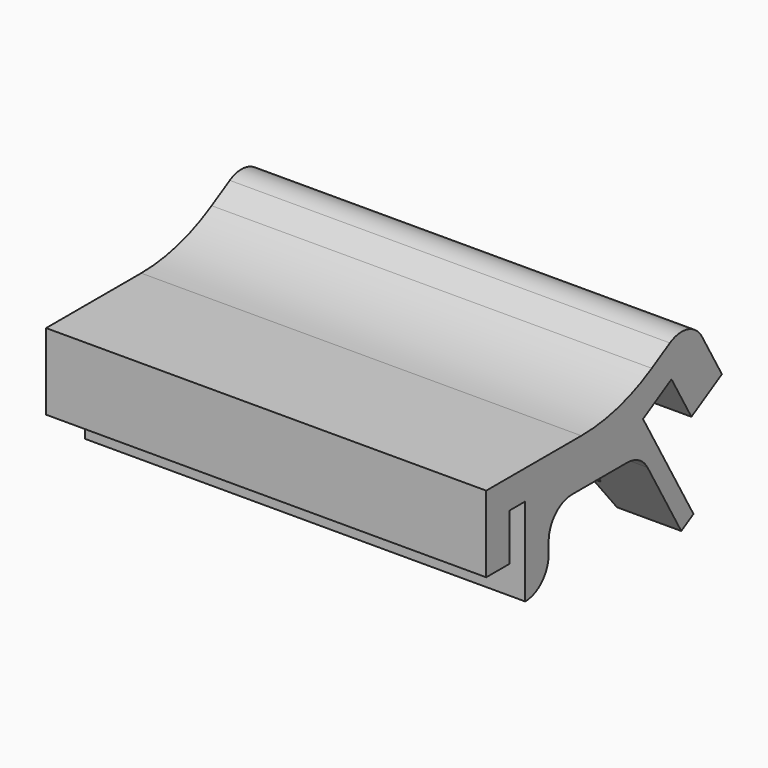
from build123d import *

# Parameters (mm, degrees)
F1_DEPTH      = 75
F2_W          = 3.3
F2_H          = 5
F3_DEPTH      = 75
F5_DEPTH      = 3
F6_ANGLE      = -30
F7_W          = 15
F7_H          = 8
F8_DEPTH      = 75
F9_R          = 5
F10_T1_DEPTH  = 75
F10_T6_DEPTH  = 82.2168783649
F10_T11_DEPTH = 82.2168783649
F10_T17_DEPTH = 89.4337567297
F10_T23_DEPTH = 82.2168783649
F10_T25_DEPTH = 100
F11_R         = 30


# Not quite as in the source:
# - a fillet or chamfer that OpenCascade refuses, or shapes differently, is made with other operations: its cross-section is extruded or revolved along the edge and cut away or added


with BuildPart() as f1:
    # F0 (on Right) → F1 (new body)
    with BuildSketch(Plane.YZ):
        Polygon((3, 13.5), (0, 13.5), (0, -13), (3, -13), (3, 8.5), (10, 8.5), (10, 0), (17.5, 0), (17.5, 13.5), (10, 13.5), align=None)
    extrude(amount=F1_DEPTH)

    # F4 (on Front) → F5 (cut, through all)
    with BuildSketch(Plane.XZ):
        Polygon((11.5, 2.5), (11.5, -7.5), (13, -7.5), (11.1212156062, -13), (33, -13), (33, -7.4999375637), (33, 2.5), align=None)
        Polygon((63.5, 2.5), (42, 2.5), (42, -7.4999375637), (42, -13), (64.044855535, -13), (62, -7.5), (63.5, -7.5), align=None)
    extrude(amount=-F5_DEPTH, mode=Mode.SUBTRACT)


with BuildPart() as f3:
    # F2 (on Right) → F3 (new body)
    with BuildSketch(Plane.YZ):
        Polygon((-23.3, 13.5), (-28.3, 13.5), (-28.3, 0.5), (-23.3, 0.5), (-23.3, 8.5), align=None)
        with Locations((-21.65, 11)):
            Rectangle(F2_W, F2_H)
        Polygon((-15, 13.5), (-20, 13.5), (-20, 8.5), (-20, -6.5), (-15, -6.5), align=None)
    extrude(amount=F3_DEPTH)


with BuildPart() as f1_1:
    # F6: moved
    add(f1.part.rotate(Axis((37.5, 0, 13.5), (-1, 0, 0)), F6_ANGLE))


    add(f3.part)  # F8 merges F3
    # F7 (on Right) → F8 (join)
    with BuildSketch(Plane.YZ):
        with Locations((-7.5, 9.5)):
            Rectangle(F7_W, F7_H)
        Polygon((5.764299538, 5.5), (0, 13.5), (0, 5.5), align=None)
    extrude(amount=F8_DEPTH)

    # F9
    f9_edges = [f1_1.edges().sort_by_distance(p)[0] for p in [
        (37.5, 15.155445, 22.25),
    ]]
    fillet(f9_edges, radius=F9_R)

    # F10: fillet of radius 5 on 3 edges, made by hand

    # F10_s2 → F10_t1 (join)
    with BuildSketch(Plane.YZ):
        with BuildLine():
            ThreePointArc((-10, 5.5), (-13.5355339059, 4.0355339059), (-15, 0.5))
            Line((-15, 0.5), (-15, 5.5))
            Line((-15, 5.5), (-10, 5.5))
        make_face()
    extrude(amount=F10_T1_DEPTH)


with BuildPart() as f10_tool4:
    # F10_s5 → F10_t6 (new body)
    with BuildSketch(Plane.YZ):
        with BuildLine():
            ThreePointArc((6.0621778265, 3), (4.2320508076, 4.8301270189), (1.7320508076, 5.5))
            Line((1.7320508076, 5.5), (4.6188021535, 5.5))
            Line((4.6188021535, 5.5), (6.0621778265, 3))
        make_face()
    extrude(amount=F10_T6_DEPTH)

    split(bisect_by=Plane.YZ.offset(11.5), keep=Keep.BOTTOM)


with BuildPart() as f1_2:
    add(f1_1.part)

    # F10_t3: union F10_tool4
    add(f10_tool4.part)


with BuildPart() as f10_tool9:
    # F10_s10 → F10_t11 (new body)
    with BuildSketch(Plane.YZ.offset(-7.2168783649)):
        with BuildLine():
            ThreePointArc((6.0621778265, 3), (4.2320508076, 4.8301270189), (1.7320508076, 5.5))
            Line((1.7320508076, 5.5), (4.6188021535, 5.5))
            Line((4.6188021535, 5.5), (6.0621778265, 3))
        make_face()
    extrude(amount=F10_T11_DEPTH)

    split(bisect_by=Plane(origin=(0, -0.3456714755, 0.5987205584), x_dir=(1, 0, 0), z_dir=(0, -0.5, 0.8660254038)), keep=Keep.TOP)

    split(bisect_by=Plane.YZ.offset(11.5), keep=Keep.TOP)


with BuildPart() as f1_3:
    add(f1_2.part)

    # F10_t8: union F10_tool9
    add(f10_tool9.part)


with BuildPart() as f10_tool15:
    # F10_s16 → F10_t17 (new body)
    with BuildSketch(Plane.YZ.offset(-7.2168783649)):
        with BuildLine():
            ThreePointArc((6.0621778265, 3), (4.2320508076, 4.8301270189), (1.7320508076, 5.5))
            Line((1.7320508076, 5.5), (4.6188021535, 5.5))
            Line((4.6188021535, 5.5), (6.0621778265, 3))
        make_face()
    extrude(amount=F10_T17_DEPTH)

    split(bisect_by=Plane.YZ.offset(42), keep=Keep.BOTTOM)

    split(bisect_by=Plane.YZ.offset(33), keep=Keep.TOP)


with BuildPart() as f1_4:
    add(f1_3.part)

    # F10_t14: union F10_tool15
    add(f10_tool15.part)


with BuildPart() as f10_tool21:
    # F10_s22 → F10_t23 (new body)
    with BuildSketch(Plane.YZ.offset(-7.2168783649)):
        with BuildLine():
            ThreePointArc((6.0621778265, 3), (4.2320508076, 4.8301270189), (1.7320508076, 5.5))
            Line((1.7320508076, 5.5), (4.6188021535, 5.5))
            Line((4.6188021535, 5.5), (6.0621778265, 3))
        make_face()
    extrude(amount=F10_T23_DEPTH)

    split(bisect_by=Plane.YZ.offset(63.5), keep=Keep.TOP)


with BuildPart() as f1_5:
    add(f1_4.part)

    # F10_t20: union F10_tool21
    add(f10_tool21.part)

    # F10_s26 → F10_t25 (cut)
    with BuildSketch(Plane.YZ.offset(-12.5)):
        with BuildLine():
            ThreePointArc((-15, -1.5), (-16.4644660941, -5.0355339059), (-20, -6.5))
            Line((-20, -6.5), (-15, -6.5))
            Line((-15, -6.5), (-15, -1.5))
        make_face()
    extrude(amount=F10_T25_DEPTH, mode=Mode.SUBTRACT)

    # F11
    f11_edges = [f1_5.edges().sort_by_distance(p)[0] for p in [
        (37.5, 0, 13.5),
    ]]
    fillet(f11_edges, radius=F11_R)


solid = f1_5.part
